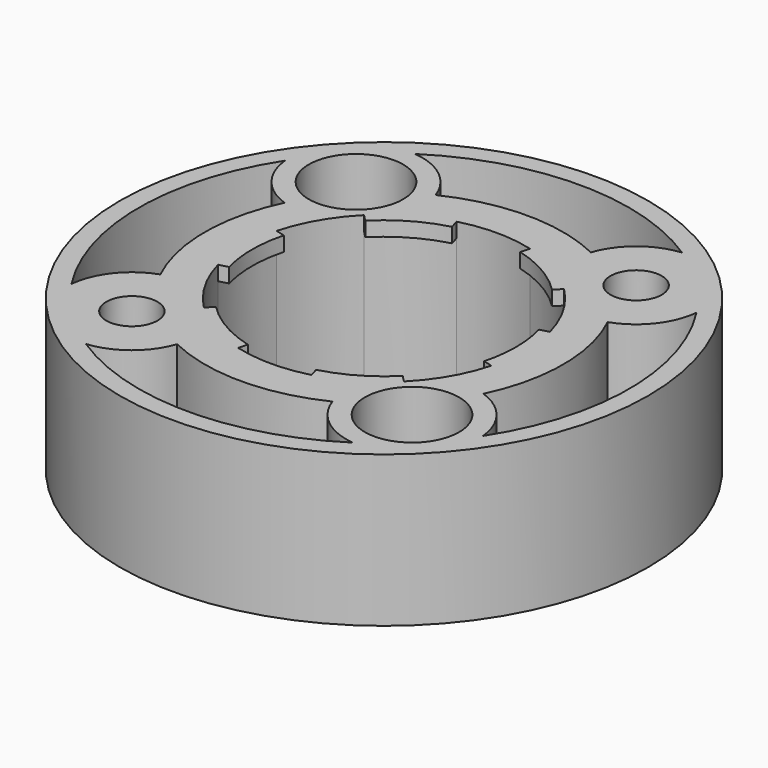
from build123d import *

# Parameters (mm, degrees)
F0_R             = 22.225
F0_R_2           = 2.15265
F1_DEPTH         = 12.7
F3_DEPTH         = 12.7
F4_COUNT         = 6
F4_ANGLE         = 300
F6_R             = 11.90625
F7_DEPTH         = 11.47445
F10_R            = 3.96875
F11_DEPTH        = 9.525
F12_R            = 3.96875
F13_DEPTH        = 9.525
F15_DEPTH        = 12.7
F15_COPIES_COUNT = 4


# Not quite as in the source:
# - a pattern or mirror of a feature is missing from the dataset's text; its kind, count and spacing are read off the source's solid


with BuildPart() as f1:
    # F0 (on Top) → F1 (new body)
    with BuildSketch(Plane.XY):
        Circle(F0_R)
        with Locations((-11.7865861589, -11.7865861589)):
            Circle(F0_R_2, mode=Mode.SUBTRACT)
        with Locations((11.7865861589, -11.7865861589)):
            Circle(F0_R_2, mode=Mode.SUBTRACT)
        with Locations((-11.7865861589, 11.7865861589)):
            Circle(F0_R_2, mode=Mode.SUBTRACT)
        with BuildLine():
            ThreePointArc((0, 11.1125), (7.8577241059, 7.8577241059), (11.1125, 0))
            ThreePointArc((11.1125, 0), (-7.8577241059, -7.8577241059), (0, 11.1125))
        make_face(mode=Mode.SUBTRACT)
        with Locations((11.7865861589, 11.7865861589)):
            Circle(F0_R_2, mode=Mode.SUBTRACT)
    extrude(amount=F1_DEPTH)

    # F2 (on face) → F3 (cut, through all)
    with BuildSketch(Plane.XY.offset(12.7)):
        with BuildLine():
            ThreePointArc((-2.8761266387, 10.7338507446), (0, 11.1125), (2.8761266387, 10.7338507446))
            Line((2.8761266387, 10.7338507446), (3.0815642558, 11.5005543693))
            ThreePointArc((3.0815642558, 11.5005543693), (0, 11.90625), (-3.0815642558, 11.5005543693))
            Line((-3.0815642558, 11.5005543693), (-2.8761266387, 10.7338507446))
        make_face()
    f3 = extrude(amount=-F3_DEPTH, mode=Mode.SUBTRACT)

    # F4: F3 ×6 about axis
    f4_axis = Axis((0, 0, 0), (0, 0, -1))
    for i in range(1, F4_COUNT):
        add(f3.rotate(f4_axis, i * F4_ANGLE / (F4_COUNT - 1)), mode=Mode.SUBTRACT)

    # F6 (on face) → F7 (cut, through all)
    with BuildSketch(Plane(origin=(0, 0, 0), x_dir=(1, 0, 0), z_dir=(0, 0, -1))):
        Circle(F6_R)
    extrude(amount=-F7_DEPTH, mode=Mode.SUBTRACT)

    # F10 (on face) → F11 (cut, through all)
    with BuildSketch(Plane(origin=(0, 0, 0), x_dir=(1, 0, 0), z_dir=(0, 0, -1))):
        with Locations((11.7865861589, -11.7865861589)):
            Circle(F10_R)
        with Locations((-11.7865861589, 11.7865861589)):
            Circle(F10_R)
    extrude(amount=-F11_DEPTH, mode=Mode.SUBTRACT)

    # F12 (on face) → F13 (cut, through all)
    with BuildSketch(Plane.XY.offset(12.7)):
        with Locations((-11.7865861589, 11.7865861589)):
            Circle(F12_R)
        with Locations((11.7865861589, -11.7865861589)):
            Circle(F12_R)
    extrude(amount=-F13_DEPTH, mode=Mode.SUBTRACT)

    # F14 (on face) → F15 (cut, through all)
    with BuildSketch(Plane(origin=(0, 0, 0), x_dir=(1, 0, 0), z_dir=(0, 0, -1))):
        with BuildLine():
            ThreePointArc((-11.229543123, 17.3148424047), (-8.3361072587, 16.1415958514), (-6.5322351826, 13.5931602316))
            ThreePointArc((-6.5322351826, 13.5931602316), (0, 15.08125), (6.5322351826, 13.5931602316))
            ThreePointArc((6.5322351826, 13.5931602316), (8.3361072587, 16.1415958514), (11.229543123, 17.3148424047))
            ThreePointArc((11.229543123, 17.3148424047), (0, 20.6375), (-11.229543123, 17.3148424047))
        make_face()
    f15 = extrude(amount=-F15_DEPTH, mode=Mode.SUBTRACT)

    # F15_copies: F15 ×4 about axis
    f15_copies_axis = Axis((0, 0, 0), (0, 0, 1))
    for i in range(1, F15_COPIES_COUNT):
        add(f15.rotate(f15_copies_axis, i * 360 / F15_COPIES_COUNT), mode=Mode.SUBTRACT)


solid = f1.part
